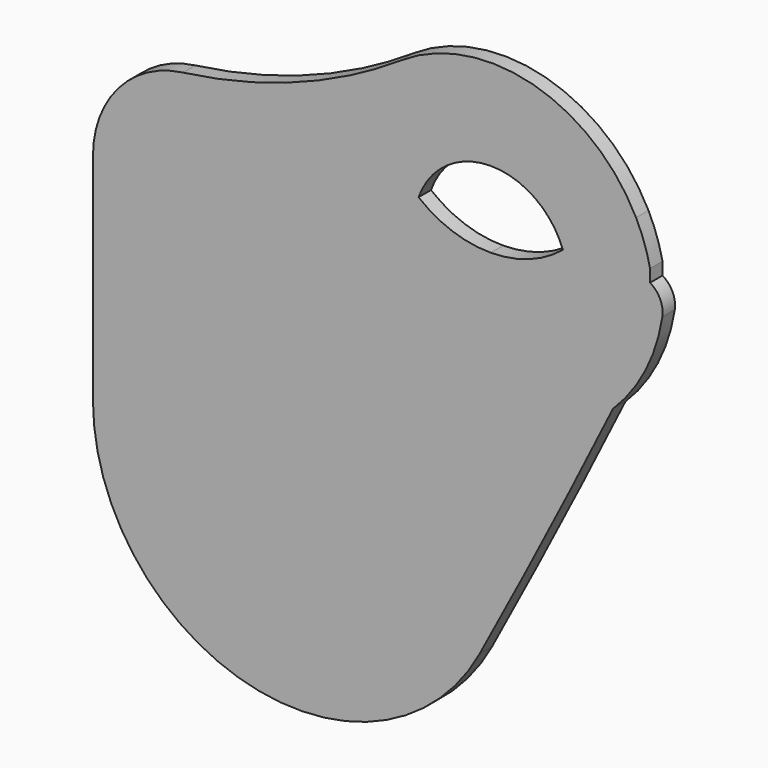
from build123d import *

# Parameters (mm, degrees)
F1_DEPTH    = 3
F2_DEPTH    = 25
F3_R        = 20
F4_R        = 100
F5_T1_DEPTH = 28.2643660281


# Not quite as in the source:
# - a fillet or chamfer that OpenCascade refuses, or shapes differently, is made with other operations: its cross-section is extruded or revolved along the edge and cut away or added


with BuildPart() as f1:
    # F0 (on Front) → F1 (new body)
    with BuildSketch(Plane.XZ):
        with BuildLine():
            ThreePointArc((-119.2295857728, 16.5976797057), (-89.2269882152, -21.8866064143), (-44.5863344816, -2.1785326218))
            ThreePointArc((-44.5863344816, -2.1785326218), (-31.5003837254, 22.7075657451), (-18.8527258188, 47.819251244))
            ThreePointArc((-18.8527258188, 47.819251244), (-11.5073907558, 58.7139707042), (-8.9261215756, 71.5975225718))
            Line((-8.9261215756, 71.5975225718), (-11.67442069, 71.5975225718))
            Line((-11.67442069, 71.5975225718), (-11.67442069, 74.0203762137))
            ThreePointArc((-11.67442069, 74.0203762137), (-12.7707106261, 77.9833199576), (-14.3762885703, 81.7686725444))
            ThreePointArc((-14.3762885703, 81.7686725444), (-44.33377908, 98.9465167224), (-71.9061774941, 78.1548738354))
            Line((-71.9061774941, 78.1548738354), (-107.2845857728, 78.1548738354))
            Line((-107.2845857728, 78.1548738354), (-119.2295857728, 78.1548738354))
            Line((-119.2295857728, 78.1548738354), (-119.2295857728, 66.2098738354))
            Line((-119.2295857728, 66.2098738354), (-119.2295857728, 16.5976797057))
        make_face()
        with BuildLine():
            ThreePointArc((-26.6928125913, 79.0930187933), (-24.6315082315, 75.5227380173), (-23.3711215756, 71.597523888))
            Line((-23.3711215756, 71.597523888), (-20.8711215756, 71.5975236602))
            ThreePointArc((-20.8711215756, 71.5975236602), (-22.8939959961, 62.4935676044), (-28.5819229469, 55.1029300277))
            ThreePointArc((-28.5819229469, 55.1029300277), (-41.6104278008, 29.1671780434), (-55.1096433175, 3.4732809051))
            ThreePointArc((-55.1096433175, 3.4732809051), (-86.3130475025, -10.3024804429), (-107.2845857728, 16.5976797057))
            Line((-107.2845857728, 16.5976797057), (-107.2845857728, 66.2098738354))
            Line((-107.2845857728, 66.2098738354), (-104.7845857728, 66.2098738354))
            Line((-104.7845857728, 66.2098738354), (-68.5864427672, 66.2098738354))
            Line((-68.5864427672, 66.2098738354), (-63.1803487139, 66.2098738354))
            ThreePointArc((-63.1803487139, 66.2098738354), (-63.6941147242, 68.8812286524), (-63.8664115811, 71.5960777945))
            Line((-63.8664115811, 71.5960777945), (-61.3664115868, 71.5962461647))
            ThreePointArc((-61.3664115868, 71.5962461647), (-46.4685424734, 86.625019162), (-26.6928125913, 79.0930187933))
        make_face(mode=Mode.SUBTRACT)
        with BuildLine():
            ThreePointArc((-32.7025071715, 52.3956462756), (-51.243606048, 52.0172813271), (-63.1803487139, 66.2098738354))
            Line((-63.1803487139, 66.2098738354), (-68.5864427672, 66.2098738354))
            Line((-68.5864427672, 66.2098738354), (-104.7845857728, 66.2098738354))
            Line((-104.7845857728, 66.2098738354), (-104.7845857728, 16.5976797057))
            ThreePointArc((-104.7845857728, 16.5976797057), (-85.7031813006, -7.8780087034), (-57.3120938901, 4.6561636023))
            ThreePointArc((-57.3120938901, 4.6561636023), (-44.8056231456, 28.4219407394), (-32.7025071715, 52.3956462756))
        make_face()
        with BuildLine():
            ThreePointArc((-61.3664115868, 71.5962461647), (-42.368127741, 52.5998806027), (-23.3711215756, 71.597523888))
            Line((-23.3711215756, 71.597523888), (-28.5062876117, 71.7030383349))
            ThreePointArc((-28.5062876117, 71.7030383348), (-35.0280474509, 67.9936357913), (-42.4162418184, 66.6868830916))
            ThreePointArc((-42.4162418184, 66.6868830916), (-49.8149115034, 67.9342855665), (-56.3664115866, 71.5913571683))
            Line((-56.3664115866, 71.5913571683), (-61.3664115868, 71.5962461647))
        make_face()
        with BuildLine():
            ThreePointArc((-55.1096433175, 3.4732809051), (-41.6104278008, 29.1671780434), (-28.5819229469, 55.1029300277))
            ThreePointArc((-28.5819229469, 55.1029300277), (-30.5643455059, 53.6307678626), (-32.7025071715, 52.3956462756))
            ThreePointArc((-32.7025071715, 52.3956462756), (-44.8056231456, 28.4219407394), (-57.3120938901, 4.6561636023))
            ThreePointArc((-57.3120938901, 4.6561636023), (-85.7031813006, -7.8780087034), (-104.7845857728, 16.5976797057))
            Line((-104.7845857728, 16.5976797057), (-104.7845857728, 66.2098738354))
            Line((-104.7845857728, 66.2098738354), (-107.2845857728, 66.2098738354))
            Line((-107.2845857728, 66.2098738354), (-107.2845857728, 16.5976797057))
            ThreePointArc((-107.2845857728, 16.5976797057), (-86.3130475025, -10.3024804429), (-55.1096433175, 3.4732809051))
        make_face()
        with BuildLine():
            ThreePointArc((-42.4162418184, 66.6868830916), (-35.0280474509, 67.9936357913), (-28.5062876117, 71.7030383348))
            ThreePointArc((-28.5062876117, 71.7030383349), (-42.4756351565, 81.447422187), (-56.3664115866, 71.5913571683))
            ThreePointArc((-56.3664115866, 71.5913571683), (-49.8149115034, 67.9342855665), (-42.4162418184, 66.6868830916))
        make_face()
        with BuildLine():
            Line((-28.5062876117, 71.7030383349), (-23.3711215756, 71.597523888))
            ThreePointArc((-23.3711215756, 71.597523888), (-24.6315082315, 75.5227380173), (-26.6928125913, 79.0930187933))
            ThreePointArc((-26.6928125913, 79.0930187933), (-46.4685424734, 86.625019162), (-61.3664115868, 71.5962461647))
            Line((-61.3664115868, 71.5962461647), (-56.3664115866, 71.5913571683))
            ThreePointArc((-56.3664115866, 71.5913571683), (-42.4756351565, 81.447422187), (-28.5062876117, 71.7030383349))
        make_face()
        with BuildLine():
            Line((-20.8711215756, 71.5975236602), (-23.3711215756, 71.597523888))
            ThreePointArc((-23.3711215756, 71.597523888), (-42.368127741, 52.5998806027), (-61.3664115868, 71.5962461647))
            Line((-61.3664115868, 71.5962461647), (-63.8664115811, 71.5960777945))
            ThreePointArc((-63.8664115811, 71.5960777945), (-63.6941147242, 68.8812286524), (-63.1803487139, 66.2098738354))
            ThreePointArc((-63.1803487139, 66.2098738354), (-51.243606048, 52.0172813271), (-32.7025071715, 52.3956462756))
            ThreePointArc((-32.7025071715, 52.3956462756), (-30.5643455059, 53.6307678626), (-28.5819229469, 55.1029300277))
            ThreePointArc((-28.5819229469, 55.1029300277), (-22.8939959961, 62.4935676044), (-20.8711215756, 71.5975236602))
        make_face()
    extrude(amount=F1_DEPTH)

    # F0 (on Front) → F2 (cut)
    with BuildSketch(Plane.XZ):
        with BuildLine():
            ThreePointArc((-42.4162418184, 66.6868830916), (-35.0280474509, 67.9936357913), (-28.5062876117, 71.7030383348))
            ThreePointArc((-28.5062876117, 71.7030383349), (-42.4756351565, 81.447422187), (-56.3664115866, 71.5913571683))
            ThreePointArc((-56.3664115866, 71.5913571683), (-49.8149115034, 67.9342855665), (-42.4162418184, 66.6868830916))
        make_face()
    extrude(amount=F2_DEPTH, mode=Mode.SUBTRACT)

    # F3
    f3_edges = [f1.edges().sort_by_distance(p)[0] for p in [
        (-119.229586, -1.5, 78.154874),
    ]]
    fillet(f3_edges, radius=F3_R)

    # F4
    f4_edges = [f1.edges().sort_by_distance(p)[0] for p in [
        (-71.906177, -1.5, 78.154874),
    ]]
    fillet(f4_edges, radius=F4_R)

    # F5: fillet of radius 5 on 1 edges, made by hand

    # F5_s2 → F5_t1 (cut)
    with BuildSketch(Plane.XZ.offset(-12.632183014)):
        with BuildLine():
            ThreePointArc((-11.67442069, 71.5975225718), (-9.7251397256, 69.4380959712), (-9.3078431517, 66.5590886613))
            ThreePointArc((-9.3078431517, 66.5590886613), (-9.0216886325, 69.0710859777), (-8.9261215756, 71.5975225718))
            Line((-8.9261215756, 71.5975225718), (-11.67442069, 71.5975225718))
        make_face()
    extrude(amount=F5_T1_DEPTH, mode=Mode.SUBTRACT)


solid = f1.part
